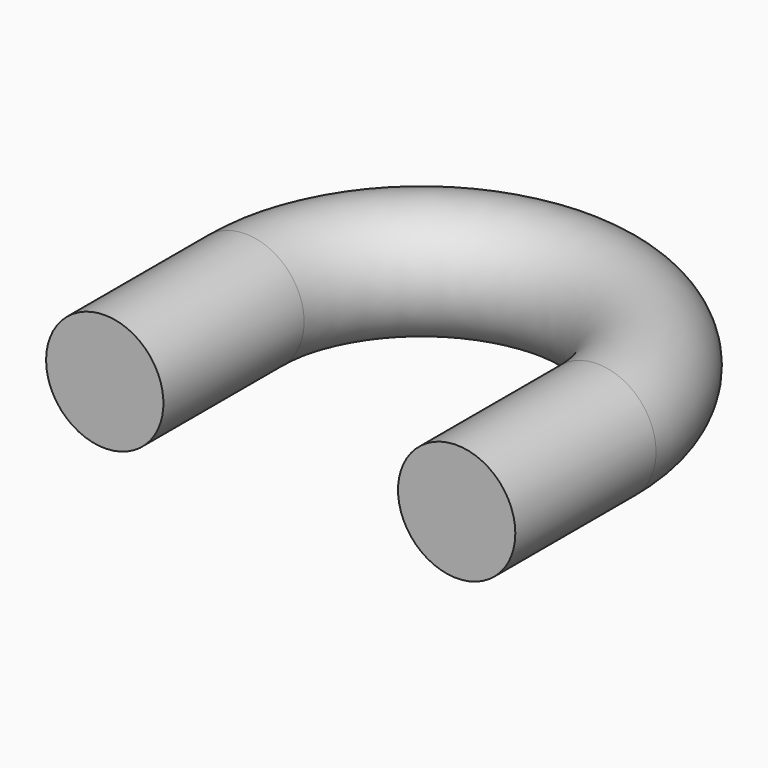
from build123d import *

# Parameters (mm, degrees)
F1_R = 12.7


with BuildPart() as f2:
    # F2: sweep along a path in F0
    with BuildLine(Plane.XY) as f2_path:
        Line((38.1, 0), (38.1, 38.1))
        ThreePointArc((38.1, 38.1), (0, 76.2), (-38.1, 38.1))
        Line((-38.1, 38.1), (-38.1, 0))
    # F1 (on Front) → F2 (sweep)
    with BuildSketch(Plane.XZ):
        with Locations((38.1, 0)):
            Circle(F1_R)
    sweep(path=f2_path.line)


solid = f2.part
